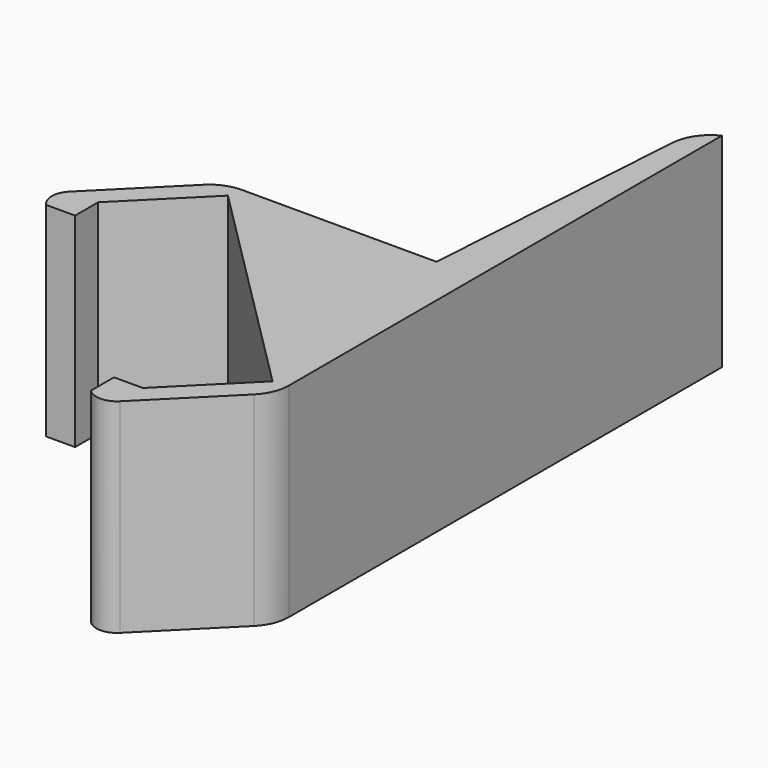
from build123d import *

# Parameters (mm, degrees)
F1_DEPTH    = 5
F2_R        = 2
F3_R        = 0.99999
F4_T1_DEPTH = 18.321255839


# Not quite as in the source:
# - a fillet or chamfer that OpenCascade refuses, or shapes differently, is made with other operations: its cross-section is extruded or revolved along the edge and cut away or added
# - a fillet or chamfer is up to 0.001 mm smaller than in the source, because OpenCascade refuses the exact size


with BuildPart() as f1:
    # F0 (on Top) → F1 (new body, symmetric)
    with BuildSketch(Plane.XY):
        Polygon((-3.2426406871, -26.7513532198), (1, -22.5087125327), (1, 4.8656561381), (0, 4.8656561381), (-1, -10.1343438619), (-11.3743686708, -10.1343438619), (-15.6170093579, -14.3769845491), (-14.2027957955, -14.3769845491), (-10.6672618896, -10.8414506431), (0.2928932188, -21.8016057515), (-3.2426406871, -25.3371396575), align=None)
        Polygon((-3.9497474683, -27.458460001), (-3.2426406871, -26.7513532198), (-4.6568542495, -26.7513532198), align=None)
        Polygon((-4.6568542495, -26.7513532198), (-3.2426406871, -26.7513532198), (-3.2426406871, -25.3371396575), align=None)
        Polygon((-4.6568542495, -25.3371396575), (-4.6568542495, -26.7513532198), (-3.2426406871, -25.3371396575), align=None)
        Polygon((-15.6170093579, -15.7911981114), (-15.6170093579, -14.3769845491), (-16.3241161391, -15.0840913303), align=None)
        Polygon((-14.2027957955, -14.3769845491), (-15.6170093579, -14.3769845491), (-15.6170093579, -15.7911981114), align=None)
        Polygon((-14.2027957955, -15.7911981114), (-14.2027957955, -14.3769845491), (-15.6170093579, -15.7911981114), align=None)
    extrude(amount=F1_DEPTH, both=True)

    # F2
    f2_edges = [f1.edges().sort_by_distance(p)[0] for p in [
        (-11.374369, -10.134344, 0),
        (1, -22.508713, 0),
    ]]
    fillet(f2_edges, radius=F2_R)

    # F3 (radius 1 in the source; OpenCascade refuses exactly that, so slightly less here)
    f3_edges = [f1.edges().sort_by_distance(p)[0] for p in [
        (-16.324116, -15.084091, 0),
        (-3.949747, -27.45846, 0),
    ]]
    fillet(f3_edges, radius=F3_R)

    # F4: fillet of radius 2 on 1 edges, made by hand

    # F4_s2 → F4_t1 (cut)
    with BuildSketch(Plane.XY.offset(-9.1606279195)):
        with BuildLine():
            ThreePointArc((1, 4.8656561381), (0.2224588554, 4.1839894082), (-0.1107043409, 3.2050910239))
            Line((-0.1107043409, 3.2050910239), (0, 4.8656561381))
            Line((0, 4.8656561381), (1, 4.8656561381))
        make_face()
    extrude(amount=F4_T1_DEPTH, mode=Mode.SUBTRACT)


solid = f1.part
